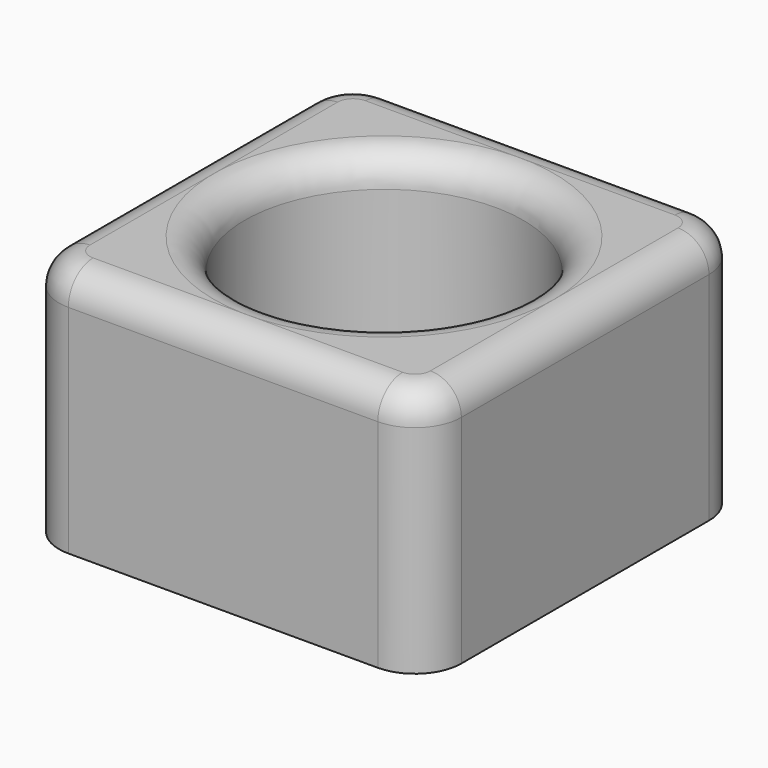
from build123d import *

# Parameters (mm, degrees)
F0_W     = 26
F0_H     = 26
F1_DEPTH = 16
F2_R     = 9
F3_DEPTH = 13.5
F4_R     = 1.65
F4_R_2   = 3.1
F5_DEPTH = 13
F6_R     = 3
F7_R     = 1.99999


# Not quite as in the source:
# - a fillet or chamfer is up to 0.001 mm smaller than in the source, because OpenCascade refuses the exact size


with BuildPart() as f1:
    # F0 (on Top) → F1 (new body)
    with BuildSketch(Plane.XY):
        Rectangle(F0_W, F0_H)
    extrude(amount=F1_DEPTH)

    # F2 (on face) → F3 (cut)
    with BuildSketch(Plane.XY.offset(16)):
        Circle(F2_R)
    extrude(amount=-F3_DEPTH, mode=Mode.SUBTRACT)

    # F4 (on face) → F5 (cut)
    with BuildSketch(Plane(origin=(0, 0, 0), x_dir=(1, 0, 0), z_dir=(0, 0, -1))):
        with Locations((8, -9)):
            Circle(F4_R)
        Circle(F4_R_2)
        with Locations((-8, 9)):
            Circle(F4_R)
    extrude(amount=-F5_DEPTH, mode=Mode.SUBTRACT)

    # F6
    f6_edges = [f1.edges().sort_by_distance(p)[0] for p in [
        (-13, 13, 8),
        (13, 13, 8),
        (-13, -13, 8),
        (13, -13, 8),
    ]]
    fillet(f6_edges, radius=F6_R)

    # F7 (radius 2 in the source; OpenCascade refuses exactly that, so slightly less here)
    f7_edges = [f1.edges().sort_by_distance(p)[0] for p in [
        (-12.12132, -12.12132, 16),
        (-13, 0, 16),
        (-12.12132, 12.12132, 16),
        (0, 13, 16),
        (12.12132, 12.12132, 16),
        (13, 0, 16),
        (12.12132, -12.12132, 16),
        (0, -13, 16),
        (-9, 0, 16),
    ]]
    fillet(f7_edges, radius=F7_R)


solid = f1.part
